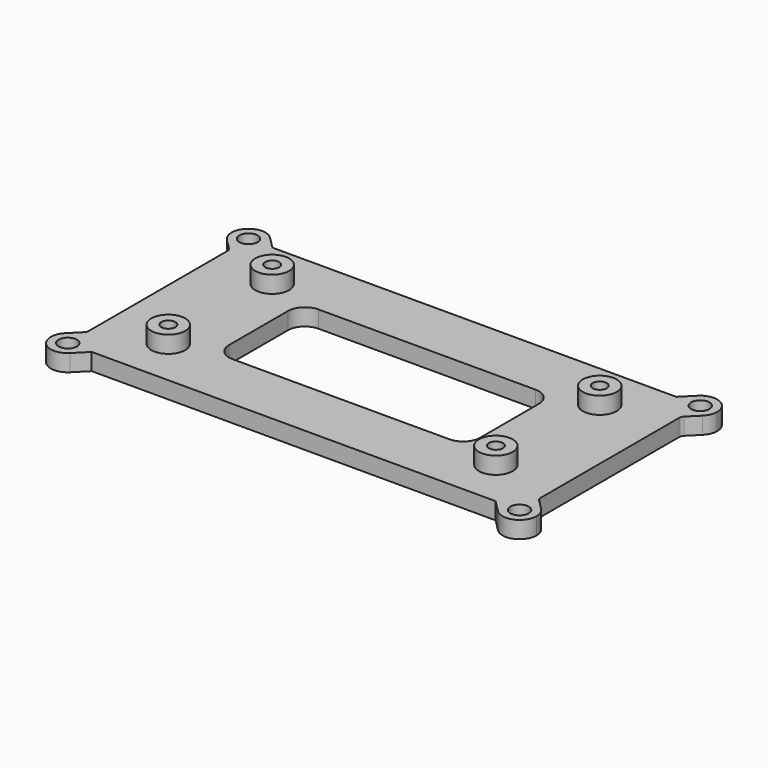
from build123d import *

# Parameters (mm, degrees)
F0_W      = 80
F0_H      = 40
F1_DEPTH  = 3
F2_R      = 3
F3_DEPTH  = 3
F5_D      = 2.5
F7_DEPTH  = 3
F9_D      = 3.25
F10_W     = 44.45
F10_H     = 19.05
F11_DEPTH = 6.001
F12_R     = 3
F13_R     = 1


# Not quite as in the source:
# - a pattern or mirror of a feature is missing from the dataset's text; its kind, count and spacing are read off the source's solid
# - a feature names something its author has since deleted; it is built from what else it names


with BuildPart() as f1:
    # F0 (on Top) → F1 (new body)
    with BuildSketch(Plane.XY):
        Rectangle(F0_W, F0_H)
    extrude(amount=F1_DEPTH)

    # F2 (on face) → F3 (join)
    with BuildSketch(Plane.XY.offset(3)):
        with Locations((-29, 11.5)):
            Circle(F2_R)
        with Locations((29, 11.5)):
            Circle(F2_R)
        with Locations((29, -11.5)):
            Circle(F2_R)
        with Locations((-29, -11.5)):
            Circle(F2_R)
    extrude(amount=F3_DEPTH)

    # F5 (through all)
    with Locations(Plane.XY.offset(6)):
        with Locations((-29, 11.5), (29, 11.5), (29, -11.5), (-29, -11.5)):
            Hole(F5_D / 2)

    # F6 (on face) → F7 (join)
    with BuildSketch(Plane(origin=(0, 0, 0), x_dir=(1, 0, 0), z_dir=(0, 0, -1))):
        with BuildLine():
            ThreePointArc((42.1213203436, 17.8786796564), (42.7716385975, 18.8519497029), (43, 20))
            ThreePointArc((43, 20), (41.1480502971, 22.7716385975), (37.8786796564, 22.1213203436))
            ThreePointArc((37.8786796564, 22.1213203436), (37.2283614025, 21.1480502971), (37, 20))
            Line((37, 20), (40, 20))
            Line((40, 20), (40, 17))
            ThreePointArc((40, 17), (41.1480502971, 17.2283614025), (42.1213203436, 17.8786796564))
        make_face()
        with BuildLine():
            ThreePointArc((37, 20), (37.2283614025, 21.1480502971), (37.8786796564, 22.1213203436))
            Line((37.8786796564, 22.1213203436), (35.7573593129, 20))
            Line((35.7573593129, 20), (37, 20))
        make_face()
        with BuildLine():
            Line((40, 15.7573593129), (42.1213203436, 17.8786796564))
            ThreePointArc((42.1213203436, 17.8786796564), (41.1480502971, 17.2283614025), (40, 17))
            Line((40, 17), (40, 15.7573593129))
        make_face()
        with BuildLine():
            Line((-37, 20), (-35.7573593129, 20))
            Line((-35.7573593129, 20), (-37.8786796564, 22.1213203436))
            ThreePointArc((-37.8786796564, 22.1213203436), (-37.2283614025, 21.1480502971), (-37, 20))
        make_face()
        with BuildLine():
            Line((42.1213203436, -17.8786796564), (40, -15.7573593129))
            Line((40, -15.7573593129), (40, -17))
            ThreePointArc((40, -17), (41.1480502971, -17.2283614025), (42.1213203436, -17.8786796564))
        make_face()
        with BuildLine():
            ThreePointArc((-37, 20), (-37.2283614025, 21.1480502971), (-37.8786796564, 22.1213203436))
            ThreePointArc((-37.8786796564, 22.1213203436), (-42.1213203436, 22.1213203436), (-42.1213203436, 17.8786796564))
            ThreePointArc((-42.1213203436, 17.8786796564), (-41.1480502971, 17.2283614025), (-40, 17))
            Line((-40, 17), (-40, 20))
            Line((-40, 20), (-37, 20))
        make_face()
        with BuildLine():
            ThreePointArc((43, -20), (42.7716385975, -18.8519497029), (42.1213203436, -17.8786796564))
            ThreePointArc((42.1213203436, -17.8786796564), (41.1480502971, -17.2283614025), (40, -17))
            Line((40, -17), (40, -20))
            Line((40, -20), (37, -20))
            ThreePointArc((37, -20), (37.2283614025, -21.1480502971), (37.8786796564, -22.1213203436))
            ThreePointArc((37.8786796564, -22.1213203436), (41.1480502971, -22.7716385975), (43, -20))
        make_face()
        with BuildLine():
            ThreePointArc((-40, 17), (-41.1480502971, 17.2283614025), (-42.1213203436, 17.8786796564))
            Line((-42.1213203436, 17.8786796564), (-40, 15.7573593129))
            Line((-40, 15.7573593129), (-40, 17))
        make_face()
        with BuildLine():
            ThreePointArc((37.8786796564, -22.1213203436), (37.2283614025, -21.1480502971), (37, -20))
            Line((37, -20), (35.7573593129, -20))
            Line((35.7573593129, -20), (37.8786796564, -22.1213203436))
        make_face()
        with BuildLine():
            Line((-40, -17), (-40, -15.7573593129))
            Line((-40, -15.7573593129), (-42.1213203436, -17.8786796564))
            ThreePointArc((-42.1213203436, -17.8786796564), (-41.1480502971, -17.2283614025), (-40, -17))
        make_face()
        with BuildLine():
            Line((-37.8786796564, -22.1213203436), (-35.7573593129, -20))
            Line((-35.7573593129, -20), (-37, -20))
            ThreePointArc((-37, -20), (-37.2283614025, -21.1480502971), (-37.8786796564, -22.1213203436))
        make_face()
        with BuildLine():
            ThreePointArc((-40, -17), (-41.1480502971, -17.2283614025), (-42.1213203436, -17.8786796564))
            ThreePointArc((-42.1213203436, -17.8786796564), (-42.1213203436, -22.1213203436), (-37.8786796564, -22.1213203436))
            ThreePointArc((-37.8786796564, -22.1213203436), (-37.2283614025, -21.1480502971), (-37, -20))
            Line((-37, -20), (-40, -20))
            Line((-40, -20), (-40, -17))
        make_face()
    extrude(amount=-F7_DEPTH)

    # F9 (through all)
    with Locations(Plane(origin=(0, 0, 0), x_dir=(1, 0, 0), z_dir=(0, 0, -1))):
        with Locations((-40, 20), (-40, -20), (40, -20)):
            f9 = Hole(F9_D / 2)

    # F9_copies: F9 across plane
    add(f9.mirror(Plane(origin=(0, 0, 0), x_dir=(0, 0, 1), z_dir=(1, 0, 0))), mode=Mode.SUBTRACT)

    # F10 (on face) → F11 (cut, through all)
    with BuildSketch(Plane(origin=(0, 0, 0), x_dir=(1, 0, 0), z_dir=(0, 0, -1))):
        Rectangle(F10_W, F10_H)
    extrude(amount=-F11_DEPTH, mode=Mode.SUBTRACT)

    # F12
    f12_edges = [f1.edges().sort_by_distance(p)[0] for p in [
        (-22.225, 9.525, 1.5),
        (22.225, -9.525, 1.5),
        (-22.225, -9.525, 1.5),
        (22.225, 9.525, 1.5),
    ]]
    fillet(f12_edges, radius=F12_R)

    # F13
    f13_edges = [f1.edges().sort_by_distance(p)[0] for p in [
        (40, 15.757359, 1.5),
        (-40, 15.757359, 1.5),
        (40, -15.757359, 1.5),
        (-40, -15.757359, 1.5),
    ]]
    fillet(f13_edges, radius=F13_R)


solid = f1.part
